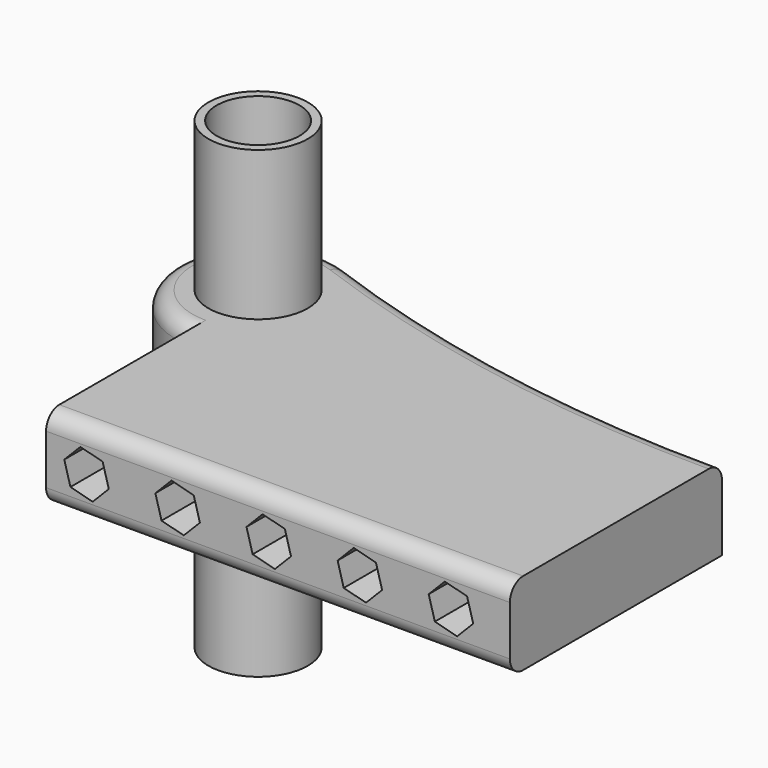
from build123d import *

# Parameters (mm, degrees)
F1_DEPTH = 25
F2_DEPTH = 70
F4_DEPTH = 120
F5_R     = 5
F6_T     = -2.5


with BuildPart() as f1:
    # F0 (on Top) → F1 (new body)
    with BuildSketch(Plane.XY):
        with BuildLine():
            Line((-70, -40), (70, -40))
            Line((70, -40), (70, 40))
            Line((70, 40), (-45.1792724346, 40))
            ThreePointArc((-45.1792724346, 40), (-52.4490952245, 22.4490952245), (-70, 15.1792724346))
            Line((-70, 15.1792724346), (-70, -40))
        make_face()
        with BuildLine():
            ThreePointArc((-61.4672239767, 63.3079439293), (-94.4396055948, 44.3329199448), (-70, 15.1792724346))
            Line((-70, 15.1792724346), (-70, 25))
            ThreePointArc((-70, 25), (-80.6066017178, 50.6066017178), (-55, 40))
            Line((-55, 40), (-45.1792724346, 40))
            ThreePointArc((-45.1792724346, 40), (-49.6547520791, 54.2175737703), (-61.4672239767, 63.3079439293))
        make_face()
        with BuildLine():
            Line((-45.1792724346, 40), (70, 40))
            ThreePointArc((70, 40), (3.2413091232, 45.8720687546), (-61.4672239767, 63.3079439293))
            ThreePointArc((-61.4672239767, 63.3079439293), (-49.6547520791, 54.2175737703), (-45.1792724346, 40))
        make_face()
        with BuildLine():
            Line((-70, 25), (-70, 15.1792724346))
            ThreePointArc((-70, 15.1792724346), (-52.4490952245, 22.4490952245), (-45.1792724346, 40))
            Line((-45.1792724346, 40), (-55, 40))
            ThreePointArc((-55, 40), (-59.3933982822, 29.3933982822), (-70, 25))
        make_face()
    extrude(amount=F1_DEPTH)

    # F3 (on face) → F4 (cut)
    with BuildSketch(Plane.XZ.offset(40)):
        Polygon((-55.9325095674, 5.813992337), (-51.0706130007, 10.7649557882), (-52.9273248392, 17.4509634512), (-59.6459332445, 19.186007663), (-64.5078298113, 14.2350442118), (-62.6511179727, 7.5490365488), align=None)
        Polygon((-37.0078298113, 14.2350442118), (-35.1511179727, 7.5490365488), (-28.4325095674, 5.813992337), (-23.5706130007, 10.7649557882), (-25.4273248392, 17.4509634512), (-32.1459332445, 19.186007663), align=None)
        Polygon((-9.5078298113, 14.2350442118), (-7.6511179727, 7.5490365488), (-0.9325095674, 5.813992337), (3.9293869993, 10.7649557882), (2.0726751608, 17.4509634512), (-4.6459332445, 19.186007663), align=None)
        Polygon((17.9921701887, 14.2350442118), (19.8488820273, 7.5490365488), (26.5674904326, 5.813992337), (31.4293869993, 10.7649557882), (29.5726751608, 17.4509634512), (22.8540667555, 19.186007663), align=None)
        Polygon((45.4921701887, 14.2350442118), (47.3488820273, 7.5490365488), (54.0674904326, 5.813992337), (58.9293869993, 10.7649557882), (57.0726751608, 17.4509634512), (50.3540667555, 19.186007663), align=None)
    extrude(amount=-F4_DEPTH, mode=Mode.SUBTRACT)

    # F5
    f5_edges = [f1.edges().sort_by_distance(p)[0] for p in [
        (0, -40, 25),
        (0, -40, 0),
        (3.241309, 45.872069, 25),
    ]]
    fillet(f5_edges, radius=F5_R)


with BuildPart() as f2:
    # F0 (on Top) → F2 (new body, symmetric)
    with BuildSketch(Plane.XY):
        with BuildLine():
            ThreePointArc((-55, 40), (-80.6066017178, 50.6066017178), (-70, 25))
            Line((-70, 25), (-70, 40))
            Line((-70, 40), (-55, 40))
        make_face()
        with BuildLine():
            Line((-70, 40), (-70, 25))
            ThreePointArc((-70, 25), (-59.3933982822, 29.3933982822), (-55, 40))
            Line((-55, 40), (-70, 40))
        make_face()
    extrude(amount=F2_DEPTH, both=True)

    # F6
    f6_openings = [f2.faces().sort_by_distance(p)[0] for p in [
        (-70, 40, 70),
        (-70, 40, -70),
    ]]
    offset(amount=F6_T, openings=f6_openings)


solid = Compound([f1.part, f2.part])
